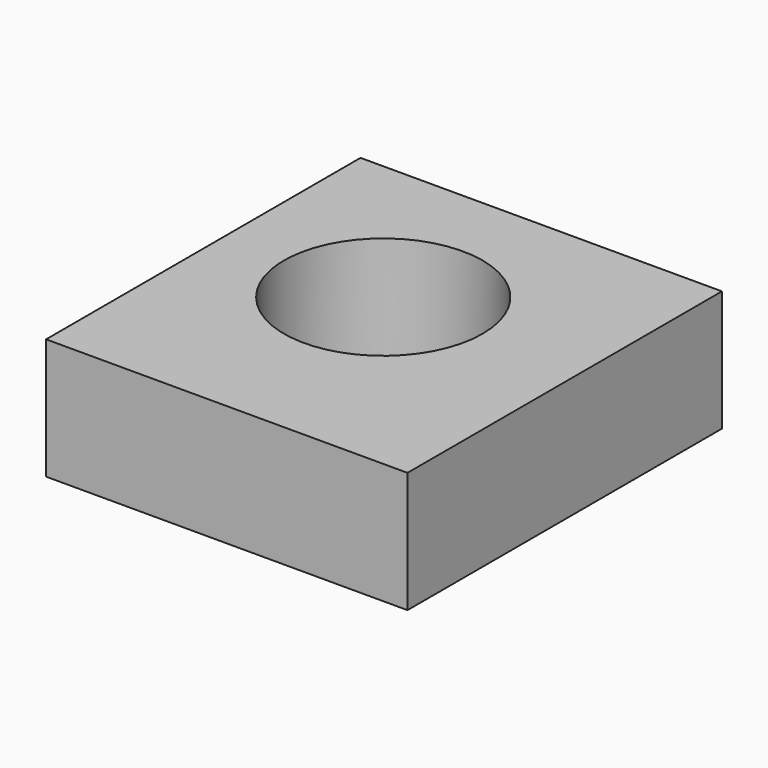
from build123d import *

# Parameters (mm, degrees)
F1_W     = 75.9237483144
F1_H     = 82.5707688928
F1_R     = 20.8624523747
F2_DEPTH = 25.4


# Not quite as in the source:
# - the program builds the solid bodies; features that only make, move or delete a surface that nothing else refers to are left out


with BuildPart() as f2:
    # F1 (on face) → F2 (new body)
    with BuildSketch(Plane.XY):
        with Locations((-7.0644952357, -4.9792416394)):
            Rectangle(F1_W, F1_H)
        with Locations((-11.2004131079, 0)):
            Circle(F1_R, mode=Mode.SUBTRACT)
    extrude(amount=F2_DEPTH)


solid = f2.part
